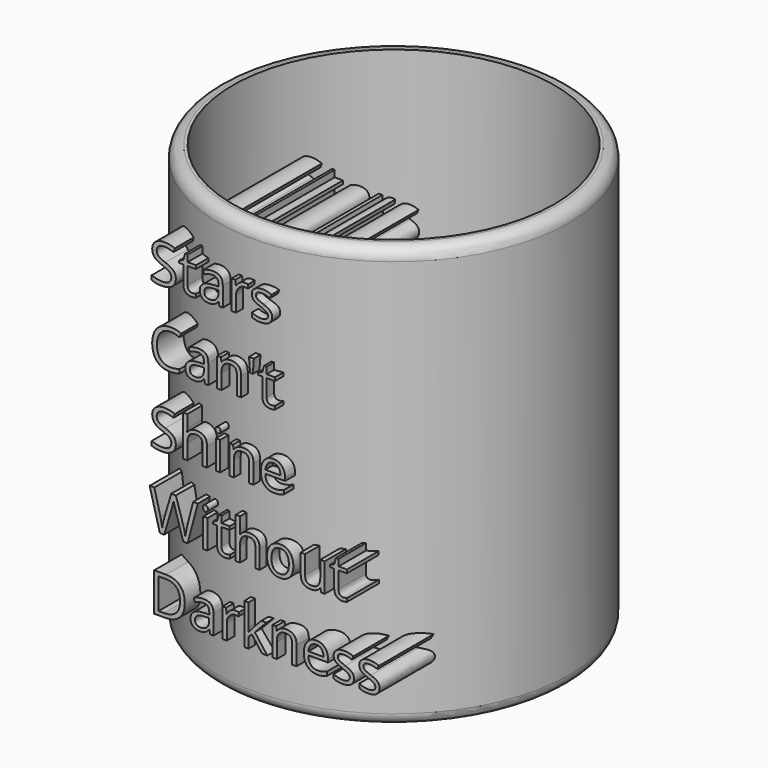
from build123d import *

# Parameters (mm, degrees)
F0_R         = 38.1
F0_R_2       = 34.925
F1_DEPTH     = 91.44
F2_R         = 34.4130561503
F3_DEPTH     = 2.54
F4_R         = 2.53999
F4_2_R       = 2.53999
F5_TEXT_SIZE = 11.6351143399
F6_DEPTH     = 39.878


# Not quite as in the source:
# - a fillet or chamfer is up to 0.001 mm smaller than in the source, because OpenCascade refuses the exact size
# - a feature of the source that left no trace in its solid (it failed there, or was rolled back) is left out
# - Text() gives the source's letters only with a copy of the font that has no kerning and outlines rounded to 1/6400 em; it was checked with that copy


with BuildPart() as f1:
    # F0 (on Top) → F1 (new body)
    with BuildSketch(Plane.XY):
        Circle(F0_R)
        Circle(F0_R_2, mode=Mode.SUBTRACT)
    extrude(amount=F1_DEPTH)

    # F4 (radius 2.54 in the source; OpenCascade refuses exactly that, so slightly less here)
    f4_edges = [f1.edges().sort_by_distance(p)[0] for p in [
        (38.1, 0, 45.72),
        (-38.1, 0, 0),
        (-38.1, 0, 91.44),
    ]]
    fillet(f4_edges, radius=F4_R)

    # F5 (on Front) → F6 (join)
    with BuildSketch(Plane.XZ):
        with Locations((-21.1939376166, 74.8141934072)):
            Text('Stars', F5_TEXT_SIZE, font='Open Sans', text_align=(TextAlign.LEFT, TextAlign.BOTTOM))
        with Locations((-21.1939376166, 58.9904379049)):
            Text("Can't", F5_TEXT_SIZE, font='Open Sans', text_align=(TextAlign.LEFT, TextAlign.BOTTOM))
        with Locations((-21.1939376166, 43.1666824026)):
            Text('Shine', F5_TEXT_SIZE, font='Open Sans', text_align=(TextAlign.LEFT, TextAlign.BOTTOM))
        with Locations((-21.1939376166, 27.3429269004)):
            Text('Without', F5_TEXT_SIZE, font='Open Sans', text_align=(TextAlign.LEFT, TextAlign.BOTTOM))
        with Locations((-21.1939376166, 11.5191713981)):
            Text('Darkness', F5_TEXT_SIZE, font='Open Sans', text_align=(TextAlign.LEFT, TextAlign.BOTTOM))
    extrude(amount=F6_DEPTH)


with BuildPart() as f3:
    # F2 (on Top) → F3 (new body)
    with BuildSketch(Plane.XY):
        Circle(F2_R)
    extrude(amount=F3_DEPTH)

    # F4#2 (radius 2.54 in the source; OpenCascade refuses exactly that, so slightly less here)
    f4_2_edges = [f3.edges().sort_by_distance(p)[0] for p in [
        (-34.413056, 0, 0),
    ]]
    fillet(f4_2_edges, radius=F4_2_R)


solid = Compound([f1.part, f3.part])
